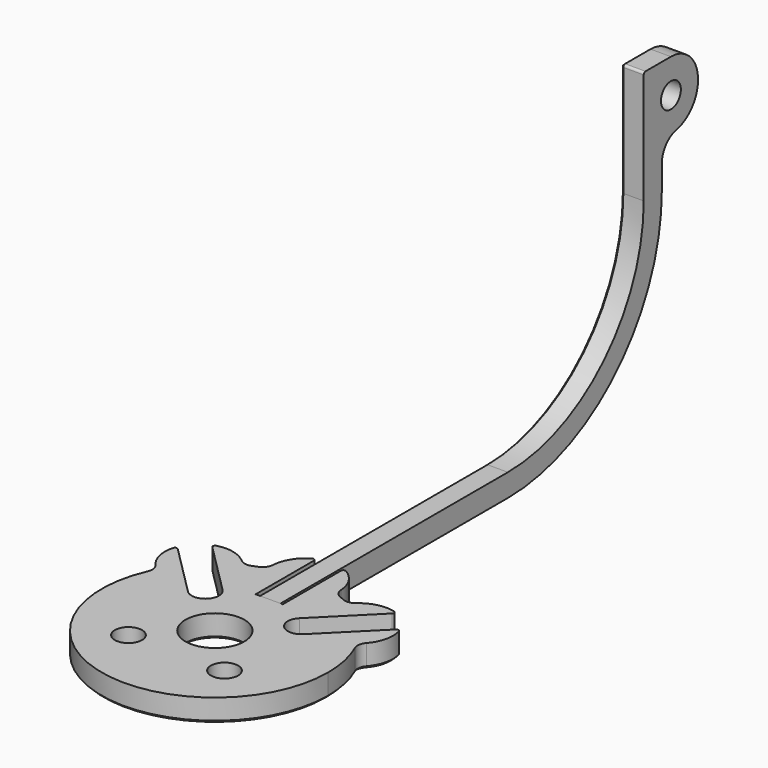
from build123d import *

# Parameters (mm, degrees)
F2_R       = 1.2
F2_R_2     = 2.6
F4_R       = 1
F5_R       = 0.2
F6_R       = 1.1
F7_DEPTH   = 1
F8_R       = 2
F9_R       = 0.2
F10_SIZE   = 0.19999
F10_2_SIZE = 0.19999


# Not quite as in the source:
# - a fillet or chamfer is up to 0.001 mm smaller than in the source, because OpenCascade refuses the exact size


with BuildPart() as f3:
    # F3: sweep along a path in F1
    with BuildLine(Plane.XZ) as f3_path:
        Line((0, 0), (0, 2))
    # F2 (on Top) → F3 (sweep)
    with BuildSketch(Plane.XY):
        with BuildLine():
            ThreePointArc((-9.8638181588, 8.166761884), (-9.9533682085, 6.2389954451), (-8.8501894784, 4.6555500422))
            ThreePointArc((-8.8501894784, 4.6555500422), (-2.3977182086, -9.7082927125), (10, 0))
            ThreePointArc((10, 0), (9.7082927125, 2.3977182086), (8.8501894784, 4.6555500422))
            ThreePointArc((8.8501894784, 4.6555500422), (9.9533682085, 6.2389954451), (9.8638181588, 8.166761884))
            Line((9.8638181588, 8.166761884), (5.0911688245, 3.3941125497))
            ThreePointArc((5.0911688245, 3.3941125497), (3.3941125497, 3.3941125497), (3.3941125497, 5.0911688245))
            Line((3.3941125497, 5.0911688245), (8.166761884, 9.8638181588))
            ThreePointArc((8.166761884, 9.8638181588), (6.2389954451, 9.9533682085), (4.6555500422, 8.8501894784))
            ThreePointArc((4.6555500422, 8.8501894784), (3.8268343237, 9.2387953251), (2.96605799, 9.55))
            ThreePointArc((2.96605799, 9.55), (2.6264581689, 11.4497301429), (1.2, 12.749545417))
            Line((1.2, 12.749545417), (1.2, 6))
            Line((1.2, 6), (-1.2, 6))
            Line((-1.2, 6), (-1.2, 12.749545417))
            ThreePointArc((-1.2, 12.749545417), (-2.6264581689, 11.4497301429), (-2.96605799, 9.55))
            ThreePointArc((-2.96605799, 9.55), (-3.8268343237, 9.2387953251), (-4.6555500422, 8.8501894784))
            ThreePointArc((-4.6555500422, 8.8501894784), (-6.2389954451, 9.9533682085), (-8.166761884, 9.8638181588))
            Line((-8.166761884, 9.8638181588), (-3.3941125497, 5.0911688245))
            ThreePointArc((-3.3941125497, 5.0911688245), (-3.3941125497, 3.3941125497), (-5.0911688245, 3.3941125497))
            Line((-5.0911688245, 3.3941125497), (-9.8638181588, 8.166761884))
        make_face()
        with Locations((-4.2426406871, -4.2426406871)):
            Circle(F2_R, mode=Mode.SUBTRACT)
        with Locations((4.2426406871, -4.2426406871)):
            Circle(F2_R, mode=Mode.SUBTRACT)
        Circle(F2_R_2, mode=Mode.SUBTRACT)
    sweep(path=f3_path.line)

    # F4
    f4_edges = [f3.edges().sort_by_distance(p)[0] for p in [
        (-8.850189, 4.65555, 1),
        (-4.65555, 8.850189, 1),
        (-2.966058, 9.55, 1),
        (2.966058, 9.55, 1),
        (4.65555, 8.850189, 1),
        (8.850189, 4.65555, 1),
    ]]
    fillet(f4_edges, radius=F4_R)

    # F5
    f5_edges = [f3.edges().sort_by_distance(p)[0] for p in [
        (-9.863818, 8.166762, 1),
        (-8.166762, 9.863818, 1),
        (-1.2, 12.749545, 1),
        (1.2, 12.749545, 1),
        (8.166762, 9.863818, 1),
        (9.863818, 8.166762, 1),
    ]]
    fillet(f5_edges, radius=F5_R)

    # F10 (size 0.2 in the source; OpenCascade refuses exactly that, so slightly less here)
    f10_edges = [f3.edges().sort_by_distance(p)[0] for p in [
        (-9.991705, 6.38559, 0),
        (-9.827424, 7.988946, 0),
        (-9.082643, 4.578766, 0),
        (-7.362704, 5.665648, 0),
        (-2.055213, -9.786526, 0),
        (-3.394113, 3.394113, 0),
        (9.786526, 2.055213, 0),
        (-5.665648, 7.362704, 0),
        (9.082643, 4.578766, 0),
        (-7.988946, 9.827424, 0),
        (9.991705, 6.38559, 0),
        (-6.38559, 9.991705, 0),
        (9.827424, 7.988946, 0),
        (-4.578766, 9.082643, 0),
        (7.362704, 5.665648, 0),
        (-3.826834, 9.238795, 0),
        (3.394113, 3.394113, 0),
        (-3.184722, 9.660075, 0),
        (5.665648, 7.362704, 0),
        (-2.549908, 11.580496, 0),
        (7.988946, 9.827424, 0),
        (-1.3, 12.598076, 0),
        (6.38559, 9.991705, 0),
        (-1.2, 9.212436, 0),
        (4.578766, 9.082643, 0),
        (0, 6, 0),
        (3.826834, 9.238795, 0),
        (1.2, 9.212436, 0),
        (3.184722, 9.660075, 0),
        (1.3, 12.598076, 0),
        (2.549908, 11.580496, 0),
        (-5.442641, -4.242641, 0),
        (3.042641, -4.242641, 0),
        (-2.6, 0, 0),
    ]]
    chamfer(f10_edges, length=F10_SIZE)


with BuildPart() as f7:
    # F6 (on Right) → F7 (new body, symmetric)
    with BuildSketch(Plane.YZ):
        with BuildLine():
            Line((6, 2), (6, 0))
            Line((6, 0), (31.1, 0))
            ThreePointArc((31.1, 0), (43.1208152802, 4.9791847198), (48.1, 17))
            Line((48.1, 17), (48.1, 21))
            Line((48.1, 21), (49.1, 21))
            ThreePointArc((49.1, 21), (52.1, 24), (49.1, 27))
            Line((49.1, 27), (46.1, 27))
            Line((46.1, 27), (46.1, 17))
            ThreePointArc((46.1, 17), (41.7066017178, 6.3933982822), (31.1, 2))
            Line((31.1, 2), (6, 2))
        make_face()
        with Locations((49.1, 24)):
            Circle(F6_R, mode=Mode.SUBTRACT)
    extrude(amount=F7_DEPTH, both=True)

    # F8
    f8_edges = [f7.edges().sort_by_distance(p)[0] for p in [
        (0, 48.1, 21),
    ]]
    fillet(f8_edges, radius=F8_R)

    # F9
    f9_edges = [f7.edges().sort_by_distance(p)[0] for p in [
        (0, 46.1, 27),
    ]]
    fillet(f9_edges, radius=F9_R)

    # F10#2 (size 0.2 in the source; OpenCascade refuses exactly that, so slightly less here)
    f10_2_edges = [f7.edges().sort_by_distance(p)[0] for p in [
        (-1, 47.7, 27),
        (-1, 46.158579, 26.941421),
        (-1, 52.084808, 24.301527),
        (-1, 46.1, 21.9),
        (-1, 48.550807, 20.365932),
        (-1, 41.706602, 6.393398),
        (-1, 48.1, 18.05051),
        (-1, 18.55, 2),
        (-1, 43.120815, 4.979185),
        (-1, 6, 1),
        (-1, 18.55, 0),
        (-1, 48, 24),
    ]]
    chamfer(f10_2_edges, length=F10_2_SIZE)


solid = Compound([f3.part, f7.part])
